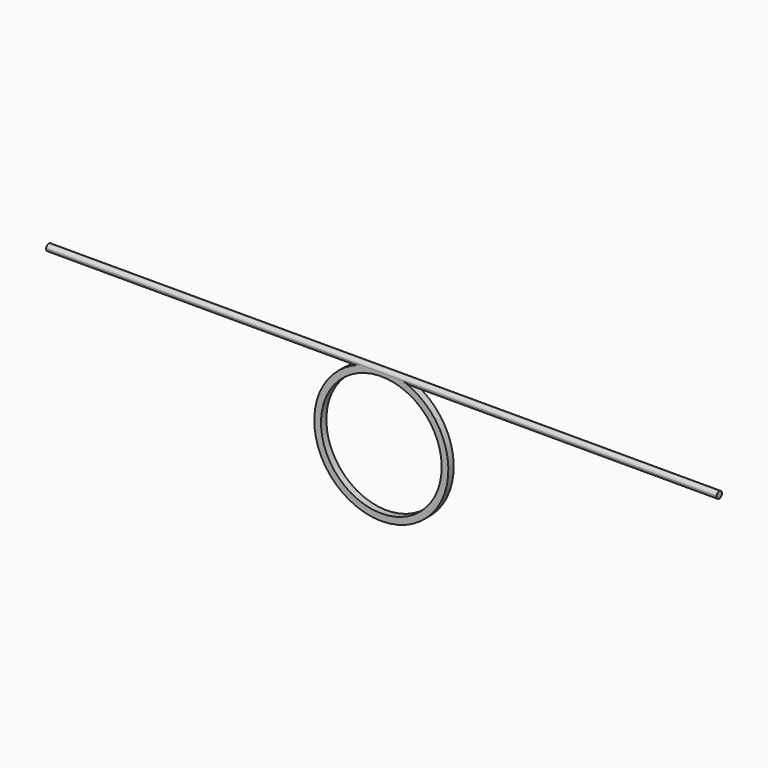
from build123d import *

# Parameters (mm, degrees)
F0_R     = 27
F1_DEPTH = 1.5
F2_R     = 1.49999


# Not quite as in the source:
# - a fillet or chamfer is up to 0.001 mm smaller than in the source, because OpenCascade refuses the exact size


with BuildPart() as f1:
    # F0 (on Front) → F1 (new body, symmetric)
    with BuildSketch(Plane.XZ):
        with BuildLine():
            Line((150, 0), (-150, 0))
            Line((-150, 0), (-150, -3))
            Line((-150, -3), (-13.0766968306, -3))
            ThreePointArc((-13.0766968306, -3), (0, -60), (13.0766968306, -3))
            Line((13.0766968306, -3), (150, -3))
            Line((150, -3), (150, 0))
        make_face()
        with Locations((0, -30)):
            Circle(F0_R, mode=Mode.SUBTRACT)
    extrude(amount=F1_DEPTH, both=True)

    # F2 (radius 1.5 in the source; OpenCascade refuses exactly that, so slightly less here)
    f2_edges = [f1.edges().sort_by_distance(p)[0] for p in [
        (-81.538348, -1.5, -3),
        (0, -1.5, 0),
        (0, 1.5, 0),
        (-81.538348, 1.5, -3),
        (81.538348, -1.5, -3),
        (81.538348, 1.5, -3),
    ]]
    fillet(f2_edges, radius=F2_R)


solid = f1.part
